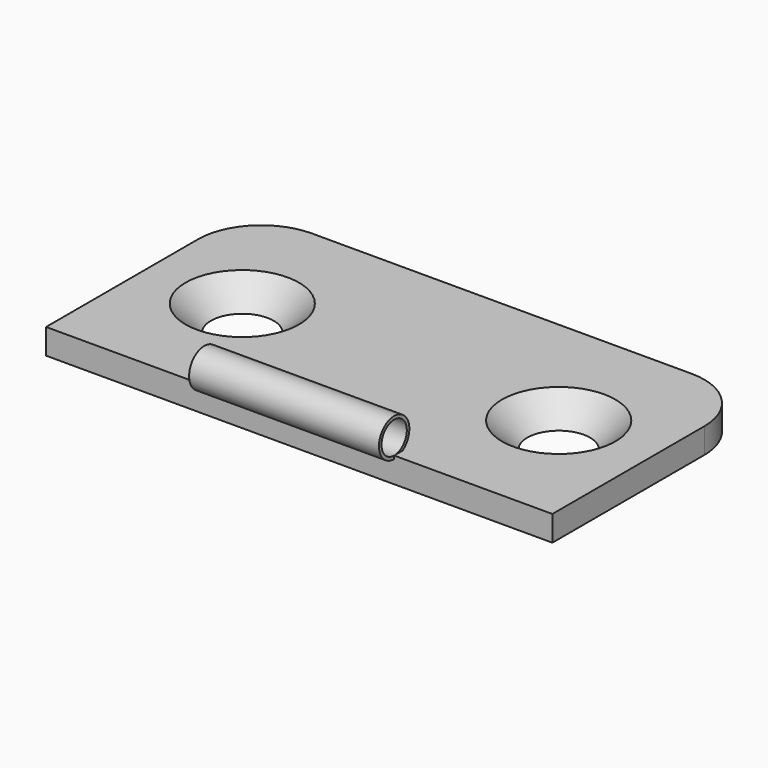
from build123d import *

# Parameters (mm, degrees)
F1_DEPTH       = 2
F3_R           = 1.5
F5_DEPTH       = 15
F6_R           = 1.25
F7_DEPTH       = 66
F9_D           = 4.4
F9_DEPTH       = 14.1
F9_CSINK_D     = 8.96
F9_CSINK_ANGLE = 90
F9_TIP         = 1.3218933619


# Not quite as in the source:
# - an extrude ends at something that could not be found from the text; its depth is read off the source's solid


with BuildPart() as f1:
    # F0 (on Top) → F1 (new body)
    with BuildSketch(Plane.XY):
        with BuildLine():
            ThreePointArc((20, 5), (18.5355339059, 8.5355339059), (15, 10))
            Line((15, 10), (-15, 10))
            ThreePointArc((-15, 10), (-18.5355339059, 8.5355339059), (-20, 5))
            Line((-20, 5), (-20, -10))
            Line((-20, -10), (20, -10))
            Line((20, -10), (20, 5))
        make_face()
    extrude(amount=F1_DEPTH)

    # F3 (on offset) → F5 (join, through all)
    with BuildSketch(Plane.YZ.offset(7.5)):
        with Locations((-10, 3.25)):
            Circle(F3_R)
    extrude(amount=-F5_DEPTH)

    # F6 (on face) → F7 (cut, through all)
    with BuildSketch(Plane.YZ.offset(20)):
        with Locations((-10, 3.25)):
            Circle(F6_R)
    extrude(amount=-F7_DEPTH, mode=Mode.SUBTRACT)

    # F9
    with Locations(Plane.XY.offset(2)):
        with Locations((-12.5, 0), (12.5, 0)):
            CounterSinkHole(F9_D / 2, F9_CSINK_D / 2, depth=F9_DEPTH, counter_sink_angle=F9_CSINK_ANGLE)
            with Locations((0, 0, -(F9_DEPTH + F9_TIP / 2))):  # 118° drill point
                Cone(0, F9_D / 2, F9_TIP, mode=Mode.SUBTRACT)


solid = f1.part
